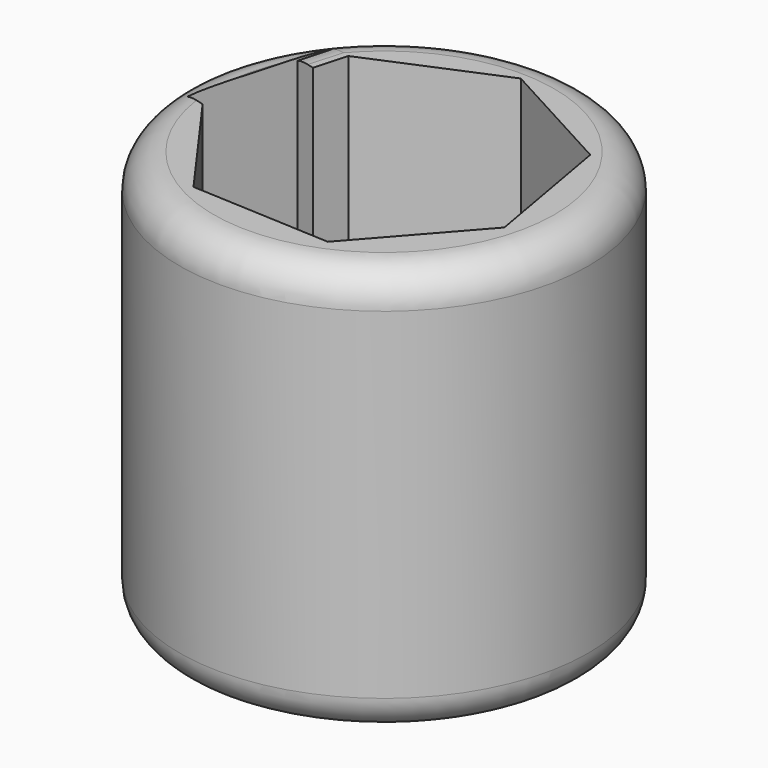
from build123d import *

# Parameters (mm, degrees)
F0_R     = 38.1
F1_DEPTH = 76.2
F3_DEPTH = 76.2
F4_R     = 6.35
F5_DEPTH = 3.81
F6_DEPTH = 6.35
F7_R     = 6.35
F8_DEPTH = 12.7


# Not quite as in the source:
# - the program builds the solid bodies; features that only make, move or delete a surface that nothing else refers to are left out


with BuildPart() as f1:
    # F0 (on Top) → F1 (new body)
    with BuildSketch(Plane.XY):
        Circle(F0_R)
    extrude(amount=F1_DEPTH)

    # F2 (on face) → F3 (cut)
    with BuildSketch(Plane.XY.offset(76.2)):
        Polygon((-22.9046876713, 20.3177796807), (-29.9596701578, -4.7970021274), (-14.7228526975, -25.9716198769), (11.3321303875, -27.2611545189), (28.5853454095, -7.6945601662), (24.0447695554, 17.9941185477), (1.1295490542, 30.4607825978), align=None)
    extrude(amount=-F3_DEPTH, mode=Mode.SUBTRACT)

    # F4
    f4_edges = [f1.edges().sort_by_distance(p)[0] for p in [
        (38.1, 0, 38.1),
        (-38.1, 0, 0),
        (-38.1, 0, 76.2),
    ]]
    fillet(f4_edges, radius=F4_R)

    # F5 (cut): a face of the model
    f5_faces = [f1.faces().sort_by_distance(p)[0] for p in [
        (-26.4321789145, 7.7603887767, 38.1),
    ]]
    extrude(f5_faces, amount=-F5_DEPTH, mode=Mode.SUBTRACT)

    # F6 (add): a face of the model
    f6_faces = [f1.faces().sort_by_distance(p)[0] for p in [
        (-24.7355489473, 20.8320861293, 38.1),
    ]]
    extrude(f6_faces, amount=F6_DEPTH)

    # F7 (on face) → F8 (cut)
    with BuildSketch(Plane(origin=(-30.1875139729, 8.4799614831, 0), x_dir=(0.2704418413, 0.9627363141, 0), z_dir=(0.9627363141, -0.2704418413, 0))):
        with Locations((-2.3566866294, 41.5975786746)):
            Circle(F7_R)
    extrude(amount=-F8_DEPTH, mode=Mode.SUBTRACT)


solid = f1.part
